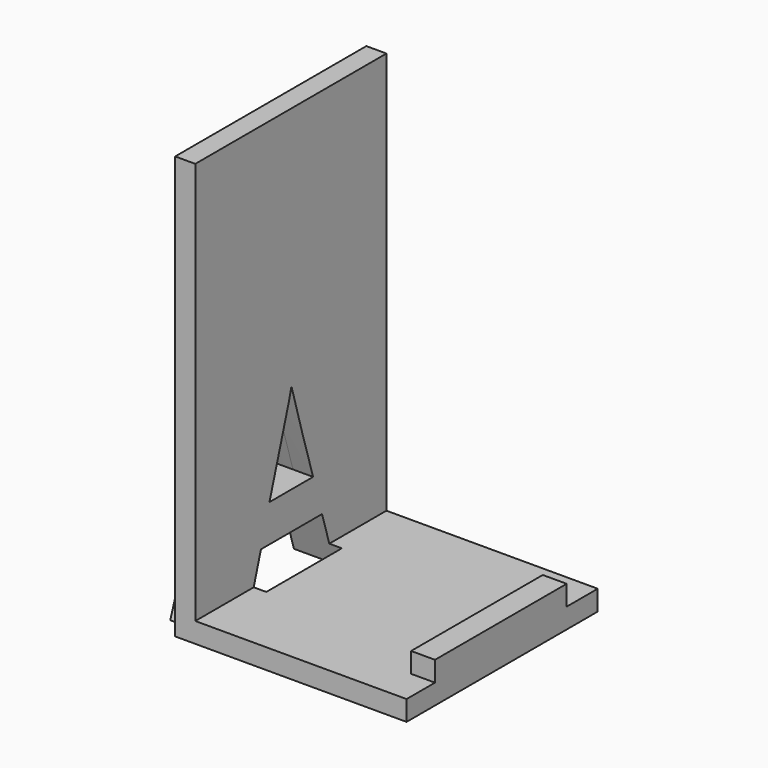
from build123d import *

# Parameters (mm, degrees)
F0_W         = 92
F0_H         = 95
F1_DEPTH     = 8
F2_W         = 8
F2_H         = 95
F3_DEPTH     = 160
F4_W         = 9.502086699
F4_H         = 65.4331929982
F5_DEPTH     = 8
F6_TEXT_SIZE = 116.6666666667
F7_DEPTH     = 8
F8_DEPTH     = 13


# Not quite as in the source:
# - Text() gives the source's letters only with a copy of the font that has no kerning and outlines rounded to 1/6400 em; it was checked with that copy


with BuildPart() as f1:
    # F0 (on Top) → F1 (new body)
    with BuildSketch(Plane.XY):
        Rectangle(F0_W, F0_H)
    extrude(amount=F1_DEPTH)

    # F2 (on face) → F3 (join)
    with BuildSketch(Plane.XY.offset(8)):
        with Locations((-42, 0)):
            Rectangle(F2_W, F2_H)
    extrude(amount=F3_DEPTH)

    # F4 (on face) → F5 (join)
    with BuildSketch(Plane.XY.offset(8)):
        with Locations((41.2489566505, -0.6576199085)):
            Rectangle(F4_W, F4_H)
    extrude(amount=F5_DEPTH)

    # F6 (on face) → F7 (join)
    with BuildSketch(Plane(origin=(-46, 0, 0), x_dir=(0, -1, 0), z_dir=(-1, 0, 0))):
        with Locations((-40.5651041667, 0)):
            Text('A', F6_TEXT_SIZE, font='Open Sans', font_style=FontStyle.BOLD, text_align=(TextAlign.LEFT, TextAlign.BOTTOM))
    extrude(amount=F7_DEPTH)

    # F8 (cut): faces of the model
    f8_faces = [f1.faces().sort_by_distance(p)[0] for p in [
        (-46, 0.2318879372, 46.4775886354),
        (-46, 0.3151041667, 9.3687753853),
    ]]
    extrude(f8_faces, amount=-F8_DEPTH, mode=Mode.SUBTRACT)


solid = f1.part
